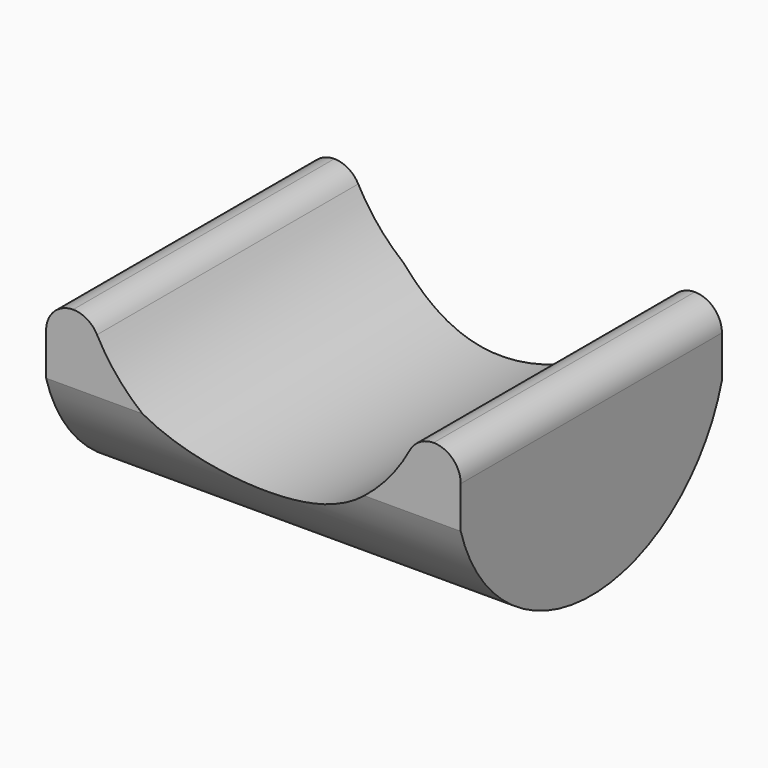
from build123d import *

# Parameters (mm, degrees)
F1_DEPTH      = 38.1
F1_DEPTH_BACK = 38.1
F3_DEPTH      = 30.48
F3_DEPTH_BACK = 30.48
F4_T1_DEPTH   = 85
F4_T3_DEPTH   = 75.73883536


# Not quite as in the source:
# - a fillet or chamfer that OpenCascade refuses, or shapes differently, is made with other operations: its cross-section is extruded or revolved along the edge and cut away or added


with BuildPart() as f1:
    # F0 (on Right) → F1 (new body, two sides)
    with BuildSketch(Plane.YZ) as f1_sk:
        with BuildLine():
            Line((-30, 12.7), (-30, 0))
            ThreePointArc((-30, 0), (0, -22.5972709807), (30, 0))
            Line((30, 0), (30, 12.7))
            Line((30, 12.7), (-30, 12.7))
        make_face()
    extrude(amount=F1_DEPTH)
    extrude(f1_sk.sketch, amount=-F1_DEPTH_BACK)

    # F2 (on Front) → F3 (cut, two sides)
    with BuildSketch(Plane.XZ) as f3_sk:
        with BuildLine():
            Line((30, 12.7), (-30, 12.7))
            ThreePointArc((-30, 12.7), (0, -7.177446186), (30, 12.7))
        make_face()
    extrude(amount=-F3_DEPTH, mode=Mode.SUBTRACT)
    extrude(f3_sk.sketch, amount=F3_DEPTH_BACK, mode=Mode.SUBTRACT)

    # F4: fillet of radius 5 on 4 edges, made by hand

    # F4_s2 → F4_t1 (cut)
    with BuildSketch(Plane.XZ.offset(-42.5)):
        with BuildLine():
            ThreePointArc((-38.1, 7.7), (-36.6355339059, 11.2355339059), (-33.1, 12.7))
            Line((-33.1, 12.7), (-38.1, 12.7))
            Line((-38.1, 12.7), (-38.1, 7.7))
        make_face()
        with BuildLine():
            ThreePointArc((33.1, 12.7), (36.6355339059, 11.2355339059), (38.1, 7.7))
            Line((38.1, 7.7), (38.1, 12.7))
            Line((38.1, 12.7), (33.1, 12.7))
        make_face()
    extrude(amount=F4_T1_DEPTH, mode=Mode.SUBTRACT)

    # F4_s4 → F4_t3 (cut)
    with BuildSketch(Plane.XZ.offset(-37.86941768)):
        with BuildLine():
            ThreePointArc((-28.7371736927, 10.0551360984), (-30.5763550564, 11.988104505), (-33.147767072, 12.7))
            Line((-33.147767072, 12.7), (-30, 12.7))
            ThreePointArc((-30, 12.7), (-29.3983455251, 11.3633593626), (-28.7371736927, 10.0551360984))
        make_face()
        with BuildLine():
            ThreePointArc((28.7371736927, 10.0551360984), (30.5763550564, 11.988104505), (33.147767072, 12.7))
            Line((33.147767072, 12.7), (30, 12.7))
            ThreePointArc((30, 12.7), (29.3983455251, 11.3633593626), (28.7371736927, 10.0551360984))
        make_face()
    extrude(amount=F4_T3_DEPTH, mode=Mode.SUBTRACT)


solid = f1.part
